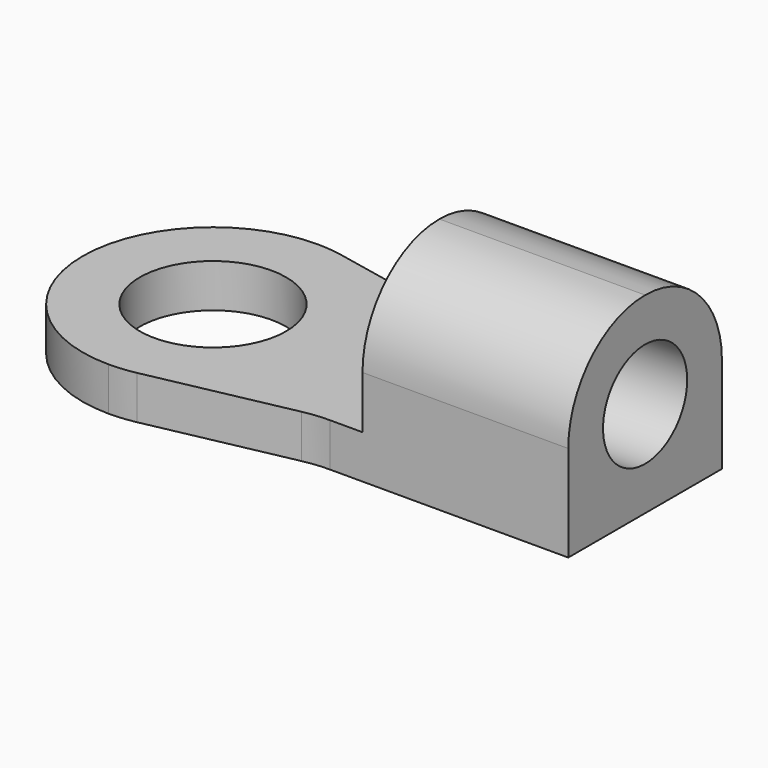
from build123d import *

# Parameters (mm, degrees)
F0_R     = 1.6
F1_DEPTH = 0.95
F2_W     = 4.5
F2_H     = 4.2
F3_DEPTH = 3.25
F4_R     = 2.09999
F5_R     = 1.15
F6_DEPTH = 25


# Not quite as in the source:
# - a fillet or chamfer is up to 0.001 mm smaller than in the source, because OpenCascade refuses the exact size


with BuildPart() as f1:
    # F0 (on Top) → F1 (new body)
    with BuildSketch(Plane.XY):
        with BuildLine():
            Line((7.088922101, 0.75), (12.3, 0.75))
            Line((12.3, 0.75), (12.3, 4.95))
            Line((12.3, 4.95), (7.088922101, 4.95))
            ThreePointArc((7.088922101, 4.95), (6.8014732986, 4.9645329863), (6.5169560678, 5.0079837291))
            Line((6.5169560678, 5.0079837291), (3.4219660332, 5.6420162709))
            ThreePointArc((3.4219660332, 5.6420162709), (3.1374488024, 5.6854670137), (2.85, 5.7))
            ThreePointArc((2.85, 5.7), (0.8347456736, 4.8652543264), (0, 2.85))
            ThreePointArc((0, 2.85), (0.8347456736, 0.8347456736), (2.85, 0))
            ThreePointArc((2.85, 0), (3.1374488024, 0.0145329863), (3.4219660332, 0.0579837291))
            Line((3.4219660332, 0.0579837291), (6.5169560678, 0.6920162709))
            ThreePointArc((6.5169560678, 0.6920162709), (6.8014732986, 0.7354670137), (7.088922101, 0.75))
        make_face()
        with Locations((2.85, 2.85)):
            Circle(F0_R, mode=Mode.SUBTRACT)
    extrude(amount=F1_DEPTH)

    # F2 (on face) → F3 (join)
    with BuildSketch(Plane.XY.offset(0.95)):
        with Locations((10.05, 2.85)):
            Rectangle(F2_W, F2_H)
    extrude(amount=F3_DEPTH)

    # F4 (radius 2.1 in the source; OpenCascade refuses exactly that, so slightly less here)
    f4_edges = [f1.edges().sort_by_distance(p)[0] for p in [
        (10.05, 4.95, 4.2),
        (10.05, 0.75, 4.2),
    ]]
    fillet(f4_edges, radius=F4_R)

    # F5 (on face) → F6 (cut)
    with BuildSketch(Plane.YZ.offset(12.3)):
        with Locations((2.85, 2.1)):
            Circle(F5_R)
    extrude(amount=-F6_DEPTH, mode=Mode.SUBTRACT)


solid = f1.part
